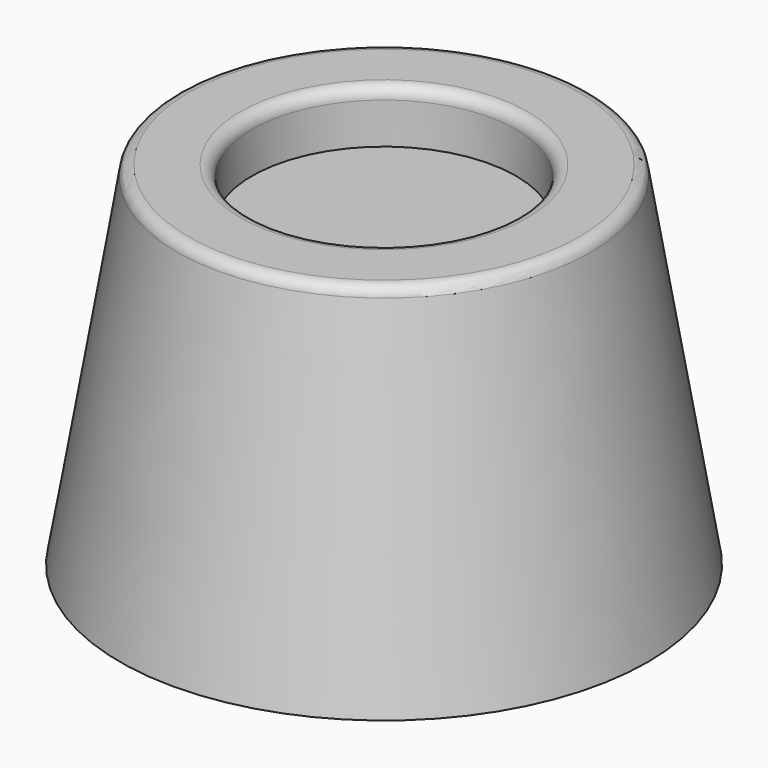
from build123d import *

# Parameters (mm, degrees)
F0_R     = 11.43
F2_R     = 8.89
F4_R     = 5.715
F5_DEPTH = 2.286
F6_R     = 0.508


with BuildPart() as f3:
    # F0 (on Top) → F3 section 0
    with BuildSketch(Plane.XY):
        Circle(F0_R)
    # F2 (on offset) → F3 section 1
    with BuildSketch(Plane.XY.offset(15.24)):
        Circle(F2_R)
    loft()

    # F4 (on face) → F5 (cut)
    with BuildSketch(Plane.XY.offset(15.24)):
        Circle(F4_R)
    extrude(amount=-F5_DEPTH, mode=Mode.SUBTRACT)

    # F6
    f6_edges = [f3.edges().sort_by_distance(p)[0] for p in [
        (-5.715, 0, 15.24),
        (-8.89, 0, 15.24),
    ]]
    fillet(f6_edges, radius=F6_R)


solid = f3.part
